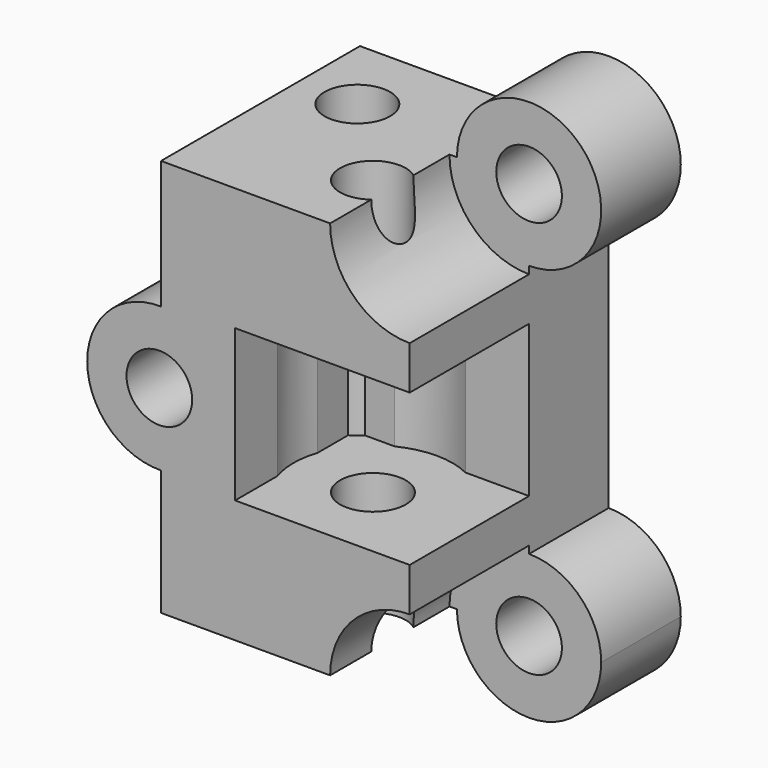
from build123d import *

# Parameters (mm, degrees)
F1_DEPTH       = 25
F3_D           = 13.2
F3_CBORE_D     = 19.25
F3_CBORE_DEPTH = 0
F5_D           = 13.2
F5_CBORE_D     = 19.25
F5_CBORE_DEPTH = 0
F6_W           = 40
F6_H           = 30.5
F7_DEPTH       = 30
F8_R           = 16
F9_DEPTH       = 30
F10_R          = 16
F11_DEPTH      = 30


with BuildPart() as f1:
    # F0 (on Front) → F1 (new body, symmetric)
    with BuildSketch(Plane.XZ):
        with BuildLine():
            Line((25, -25.5), (25, -40))
            Line((25, -40), (10.5, -40))
            ThreePointArc((10.5, -40), (25, -54.5), (39.5, -40))
            ThreePointArc((39.5, -40), (35.2530483272, -29.7469516728), (25, -25.5))
        make_face()
        with BuildLine():
            Line((10.5, -40), (25, -40))
            Line((25, -40), (25, -25.5))
            ThreePointArc((25, -25.5), (14.7469516728, -29.7469516728), (10.5, -40))
        make_face()
        with BuildLine():
            Line((-25, -40), (10.5, -40))
            ThreePointArc((10.5, -40), (14.7469516728, -29.7469516728), (25, -25.5))
            Line((25, -25.5), (25, 25.5))
            ThreePointArc((25, 25.5), (14.7469516728, 29.7469516728), (10.5, 40))
            Line((10.5, 40), (-25, 40))
            Line((-25, 40), (-25, 14.2162181315))
            ThreePointArc((-25, 14.2162181315), (-14.9640357801, 9.8540823977), (-10.8347666082, -0.279916916))
            ThreePointArc((-10.8347666082, -0.279916916), (-14.9640357801, -10.4139162298), (-25, -14.7760519636))
            Line((-25, -14.7760519636), (-25, -40))
        make_face()
        with BuildLine():
            ThreePointArc((10.5, 40), (14.7469516728, 29.7469516728), (25, 25.5))
            Line((25, 25.5), (25, 40))
            Line((25, 40), (10.5, 40))
        make_face()
        with BuildLine():
            Line((25, 40), (25, 25.5))
            ThreePointArc((25, 25.5), (35.2530483272, 29.7469516728), (39.5, 40))
            ThreePointArc((39.5, 40), (25, 54.5), (10.5, 40))
            Line((10.5, 40), (25, 40))
        make_face()
        with BuildLine():
            ThreePointArc((-25, 14.2162181315), (-39.8347666082, -0.279916916), (-25, -14.7760519636))
            Line((-25, -14.7760519636), (-25, 14.2162181315))
        make_face()
        with BuildLine():
            Line((-25, 14.2162181315), (-25, -14.7760519636))
            ThreePointArc((-25, -14.7760519636), (-14.9640357801, -10.4139162298), (-10.8347666082, -0.279916916))
            ThreePointArc((-10.8347666082, -0.279916916), (-14.9640357801, 9.8540823977), (-25, 14.2162181315))
        make_face()
    extrude(amount=F1_DEPTH, both=True)

    # F3 (through all)
    with Locations(Plane.XZ.offset(25)):
        with Locations((25, 40), (-25.3347666082, -0.279916916), (25, -40)):
            CounterBoreHole(F3_D / 2, F3_CBORE_D / 2, F3_CBORE_DEPTH)

    # F5 (through all)
    with Locations(Plane.XY.offset(40)):
        with Locations((-13, 9.3407420599), (5.0832007976, -9.3407420599)):
            CounterBoreHole(F5_D / 2, F5_CBORE_D / 2, F5_CBORE_DEPTH)

    # F6 (on face) → F7 (cut)
    with BuildSketch(Plane.XZ.offset(25)):
        with Locations((9.9, 0)):
            Rectangle(F6_W, F6_H)
    extrude(amount=-F7_DEPTH, mode=Mode.SUBTRACT)

    # F8 (on face) → F9 (cut)
    with BuildSketch(Plane.XY.offset(-15.25)):
        with Locations((5.0832007976, -9.3407420599)):
            Circle(F8_R)
    extrude(amount=F9_DEPTH, mode=Mode.SUBTRACT)

    # F10 (on face) → F11 (cut)
    with BuildSketch(Plane.XZ.offset(25)):
        with Locations((25, 40)):
            Circle(F10_R)
        with Locations((25, -40)):
            Circle(F10_R)
    extrude(amount=-F11_DEPTH, mode=Mode.SUBTRACT)


solid = f1.part
